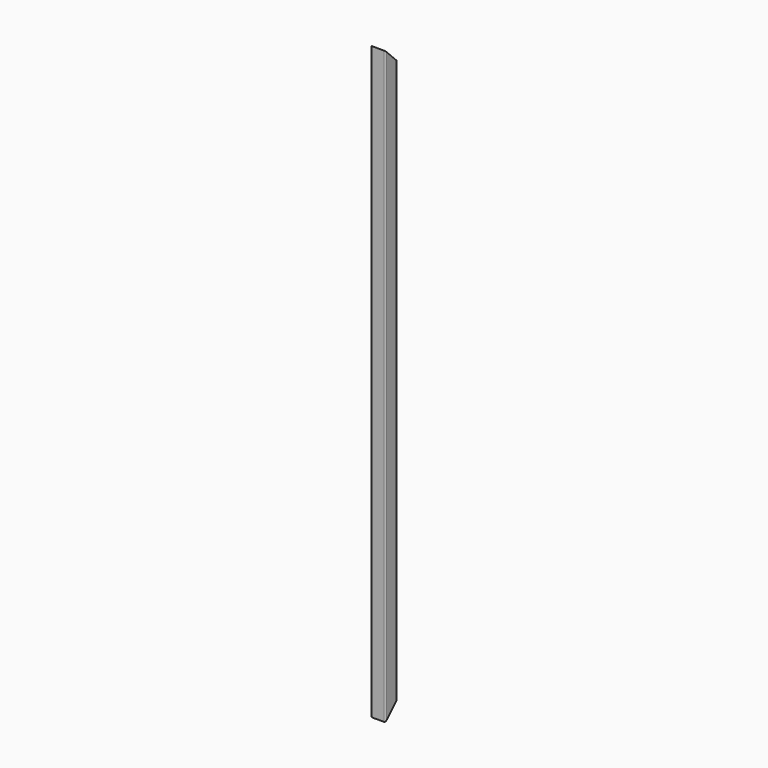
from build123d import *

# Parameters (mm, degrees)
F1_DEPTH      = 1000
F3_DEPTH      = 2000.001
F5_DEPTH      = 25.001
F5_DEPTH_BACK = 25


# Not quite as in the source:
# - a pattern or mirror of a feature is missing from the dataset's text; its kind, count and spacing are read off the source's solid


with BuildPart() as f1:
    # F0 (on Top) → F1 (new body, symmetric)
    with BuildSketch(Plane.XY):
        with BuildLine():
            ThreePointArc((25, 20), (23.5355339059, 23.5355339059), (20, 25))
            Line((20, 25), (-20, 25))
            ThreePointArc((-20, 25), (-23.5355339059, 23.5355339059), (-25, 20))
            Line((-25, 20), (-25, -20))
            ThreePointArc((-25, -20), (-23.5355339059, -23.5355339059), (-20, -25))
            Line((-20, -25), (20, -25))
            ThreePointArc((20, -25), (23.5355339059, -23.5355339059), (25, -20))
            Line((25, -20), (25, 20))
        make_face()
    extrude(amount=F1_DEPTH, both=True)

    # F2 (on face) → F3 (cut, through all)
    with BuildSketch(Plane.XY.offset(1000)):
        with BuildLine():
            ThreePointArc((-22, -20), (-21.4142135624, -21.4142135624), (-20, -22))
            Line((-20, -22), (20, -22))
            ThreePointArc((20, -22), (21.4142135624, -21.4142135624), (22, -20))
            Line((22, -20), (22, 20))
            ThreePointArc((22, 20), (21.4142135624, 21.4142135624), (20, 22))
            Line((20, 22), (-20, 22))
            ThreePointArc((-20, 22), (-21.4142135624, 21.4142135624), (-22, 20))
            Line((-22, 20), (-22, -20))
        make_face()
    extrude(amount=-F3_DEPTH, mode=Mode.SUBTRACT)

    # F4 (on Right) → F5 (cut, two sides)
    with BuildSketch(Plane.YZ) as f5_sk:
        Polygon((25, 1000), (-25, 1000), (25, 950), align=None)
    f5 = extrude(amount=-F5_DEPTH, mode=Mode.SUBTRACT) + extrude(f5_sk.sketch, amount=F5_DEPTH_BACK, mode=Mode.SUBTRACT)

    # F5_copies: F5 across plane
    add(f5.mirror(Plane(origin=(0, 0, 0), x_dir=(-1, 0, 0), z_dir=(0, 0, -1))), mode=Mode.SUBTRACT)


solid = f1.part
